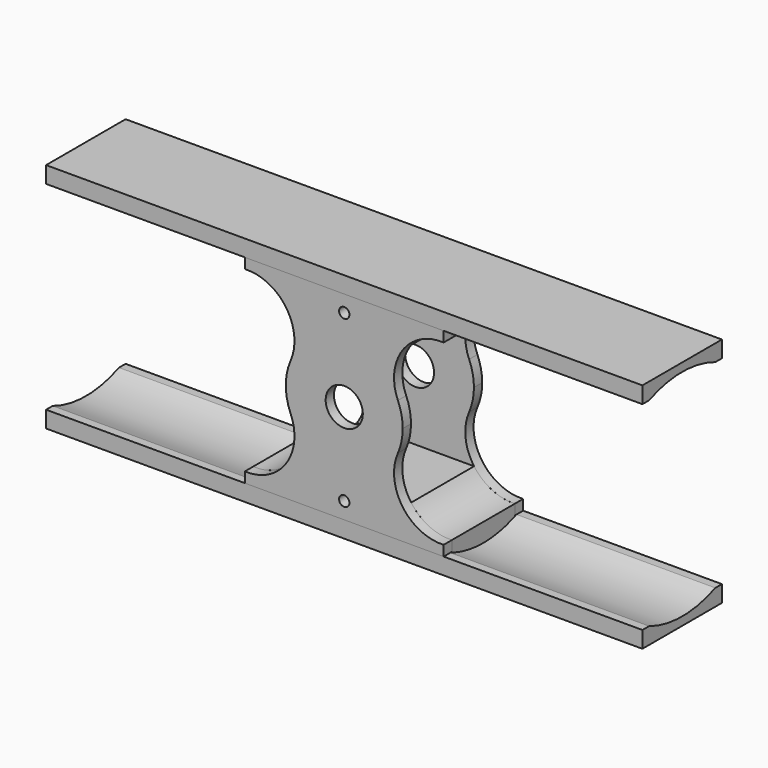
from build123d import *

# Parameters (mm, degrees)
F3_DEPTH  = 457.2
F5_R      = 7.9375
F5_R_2    = 28.4954486751
F6_DEPTH  = 15.875
F8_DEPTH  = 152.4
F9_R      = 7.9375
F10_DEPTH = 136.526


# Not quite as in the source:
# - a variable given as a bare number and used for a length is read in inches; the dataset says mm whatever the document's units were


with BuildPart() as f3:
    # F2 (on Right) → F3 (new body, symmetric)
    with BuildSketch(Plane.YZ):
        with BuildLine():
            Line((-76.2, -152.4), (-76.2, -177.8))
            Line((-76.2, -177.8), (76.2, -177.8))
            Line((76.2, -177.8), (76.2, -152.4))
            Line((76.2, -152.4), (63.5, -152.4))
            ThreePointArc((63.5, -152.4), (0, -165.1), (-63.5, -152.4))
            Line((-63.5, -152.4), (-76.2, -152.4))
        make_face()
    extrude(amount=F3_DEPTH, both=True)


with BuildPart() as f6:
    # F5 (on offset) → F6 (new body)
    with BuildSketch(Plane.XZ.offset(76.2)):
        with BuildLine():
            ThreePointArc((-82.2750366967, 35.5290866249), (0, 89.6186233985), (82.2750366967, 35.5290866249))
            ThreePointArc((82.2750366967, 35.5290866249), (89.271178874, 105.5144756245), (152.4, 136.525))
            Line((152.4, 136.525), (152.4, 152.4))
            Line((152.4, 152.4), (0, 152.4))
            Line((0, 152.4), (-152.4, 152.4))
            Line((-152.4, 152.4), (-152.4, 136.525))
            ThreePointArc((-152.4, 136.525), (-89.271178874, 105.5144756245), (-82.2750366967, 35.5290866249))
        make_face()
        with Locations((0, 127)):
            Circle(F5_R, mode=Mode.SUBTRACT)
        with BuildLine():
            ThreePointArc((82.2750366967, -35.5290866249), (87.7635265605, -18.1400403944), (89.6186233985, 0))
            ThreePointArc((89.6186233985, 0), (87.7635265605, 18.1400403944), (82.2750366967, 35.5290866249))
            ThreePointArc((82.2750366967, 35.5290866249), (0, 89.6186233985), (-82.2750366967, 35.5290866249))
            ThreePointArc((-82.2750366967, 35.5290866249), (-89.6186233985, 0), (-82.2750366967, -35.5290866249))
            ThreePointArc((-82.2750366967, -35.5290866249), (0, -89.6186233985), (82.2750366967, -35.5290866249))
        make_face()
        Circle(F5_R_2, mode=Mode.SUBTRACT)
        with BuildLine():
            ThreePointArc((152.4, -136.525), (89.271178874, -105.5144756245), (82.2750366967, -35.5290866249))
            ThreePointArc((82.2750366967, -35.5290866249), (0, -89.6186233985), (-82.2750366967, -35.5290866249))
            ThreePointArc((-82.2750366967, -35.5290866249), (-89.271178874, -105.5144756245), (-152.4, -136.525))
            Line((-152.4, -136.525), (-152.4, -152.4))
            Line((-152.4, -152.4), (0, -152.4))
            Line((0, -152.4), (152.4, -152.4))
            Line((152.4, -152.4), (152.4, -136.525))
        make_face()
        with Locations((0, -127)):
            Circle(F5_R, mode=Mode.SUBTRACT)
    extrude(amount=-F6_DEPTH)


with BuildPart() as f8:
    # F7 (on Right) → F8 (new body, symmetric)
    with BuildSketch(Plane.YZ):
        with BuildLine():
            Line((-60.325, -106.3404455781), (-60.325, -153.6844311406))
            ThreePointArc((-60.325, -153.6844311406), (0, -165.1), (60.325, -153.6844311406))
            Line((60.325, -153.6844311406), (60.325, -106.3404455781))
            Line((60.325, -106.3404455781), (-60.325, -106.3404455781))
        make_face()
    extrude(amount=F8_DEPTH, both=True)

    # F9 (on face) → F10 (cut, through all)
    with BuildSketch(Plane.XZ.offset(60.325)):
        with BuildLine():
            Line((217.5968876211, -86.5462123202), (82.2750366967, -35.5290866249))
            ThreePointArc((82.2750366967, -35.5290866249), (123.1963063092, -131.9640231824), (217.5968876211, -86.5462123202))
        make_face()
        with Locations((0, -127)):
            Circle(F9_R)
        with BuildLine():
            ThreePointArc((-217.5968876211, -86.5462123202), (-123.1963063092, -131.9640231824), (-82.2750366967, -35.5290866249))
            Line((-82.2750366967, -35.5290866249), (-217.5968876211, -86.5462123202))
        make_face()
    extrude(amount=-F10_DEPTH, mode=Mode.SUBTRACT)


with BuildPart() as f11_1:
    # F11: instance of F3
    add(f3.part.mirror(Plane.XY))


with BuildPart() as f11_2:
    # F11: instance of F8
    add(f8.part.mirror(Plane.XY))


with BuildPart() as f12_1:
    # F12: instance of F6
    add(f6.part.mirror(Plane.XZ))


solid = Compound([f3.part, f6.part, f8.part, f11_1.part, f11_2.part, f12_1.part])
